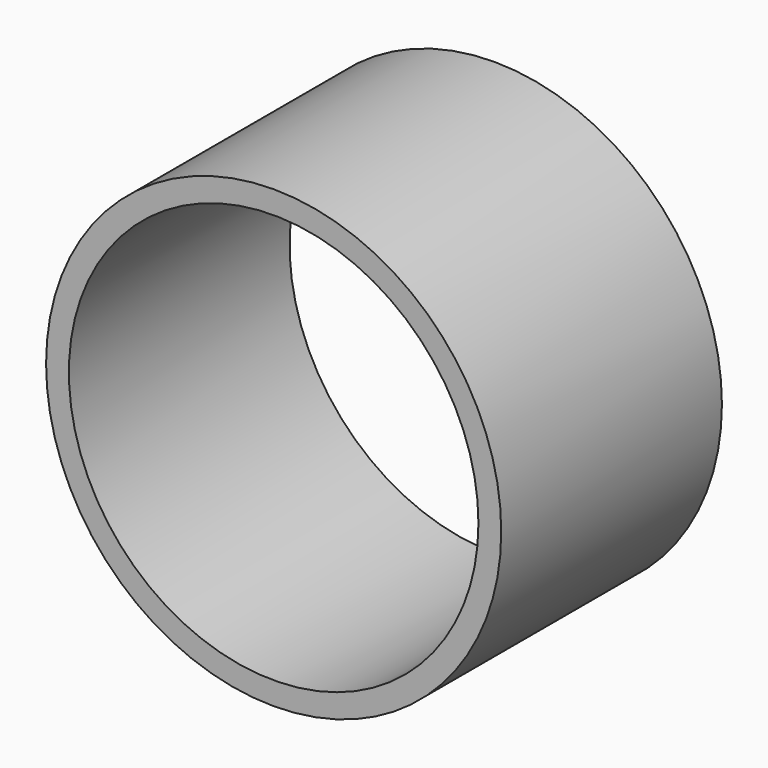
from build123d import *

# Parameters (mm, degrees)
F0_R     = 20.955
F0_R_2   = 18.8551188648
F2_DEPTH = 25.4


# Not quite as in the source:
# - the program builds the solid bodies; features that only make, move or delete a surface that nothing else refers to are left out


with BuildPart() as f2:
    # F0 (on Front) → F2 (new body)
    with BuildSketch(Plane.XZ):
        Circle(F0_R)
        Circle(F0_R_2, mode=Mode.SUBTRACT)
    extrude(amount=F2_DEPTH)


solid = f2.part
